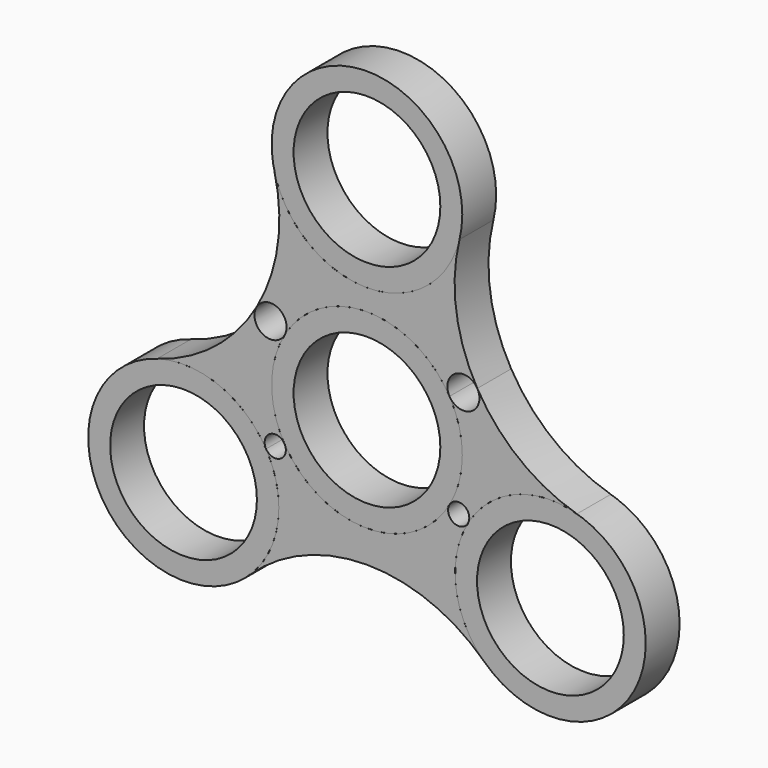
from build123d import *

# Parameters (mm, degrees)
F1_R     = 14.2875
F2_DEPTH = 6.35
F0_R     = 14.2875
F0_R_2   = 10.9982
F6_DEPTH = 25.4
F8_DEPTH = 25.4


with BuildPart() as f2:
    # F1 (on Front) → F2 (new body)
    with BuildSketch(Plane.XZ):
        with BuildLine():
            ThreePointArc((13.8718760728, 28.3289313848), (0, 17.4625), (-13.8718760728, 28.3289313848))
            ThreePointArc((-13.8718760728, 28.3289313848), (-16.5359438351, 9.5470316245), (-31.4695122777, -2.1510686152))
            ThreePointArc((-31.4695122777, -2.1510686152), (-18.912441482, -4.4535326513), (-13.2088065702, -15.875))
            ThreePointArc((-13.2088065702, -15.875), (-14.3517276668, -21.4743483284), (-17.5976362049, -26.1778627696))
            ThreePointArc((-17.5976362049, -26.1778627696), (0, -19.094063249), (17.5976362049, -26.1778627696))
            ThreePointArc((17.5976362049, -26.1778627696), (15.1229686136, -8.73125), (31.4695122777, -2.1510686152))
            ThreePointArc((31.4695122777, -2.1510686152), (16.5359438351, 9.5470316245), (13.8718760728, 28.3289313848))
        make_face()
        Circle(F1_R, mode=Mode.SUBTRACT)
    extrude(amount=F2_DEPTH)

    # F5 (on face) → F6 (cut)
    with BuildSketch(Plane.XZ.offset(6.35)):
        with BuildLine():
            ThreePointArc((12.3733379823, 7.1437499555), (15.0766559758, 6.02399903), (16.8579225203, 8.3453908122))
            ThreePointArc((16.8579225203, 8.3453908122), (16.7760327127, 8.9674057632), (16.535943943, 9.5470314377))
            ThreePointArc((16.535943943, 9.5470314377), (13.2530001547, 10.4266937926), (12.3733379823, 7.1437499555))
        make_face()
        with BuildLine():
            ThreePointArc((-16.5359438155, 9.5470316585), (-15.6562817429, 6.2640878931), (-12.3733379771, 7.1437499644))
            ThreePointArc((-12.3733379771, 7.1437499644), (-12.1332491122, 7.7233757372), (-12.0513592713, 8.3453908122))
            ThreePointArc((-12.0513592713, 8.3453908122), (-13.8326258217, 10.6667825961), (-16.5359438155, 9.5470316585))
        make_face()
    extrude(amount=-F6_DEPTH, mode=Mode.SUBTRACT)

    # F7 (on face) → F8 (cut)
    with BuildSketch(Plane.XZ.offset(6.35)):
        with BuildLine():
            ThreePointArc((15.1229686575, -8.731249924), (15.2815605457, -8.3483751917), (15.3356532851, -7.9375))
            ThreePointArc((15.3356532851, -7.9375), (14.1590284355, -6.4040927283), (12.3733378699, -7.1437501501))
            ThreePointArc((12.3733378699, -7.1437501501), (12.9544033981, -9.3123153938), (15.1229686575, -8.731249924))
        make_face()
        with BuildLine():
            ThreePointArc((-12.1606532851, -7.9375), (-12.2147460382, -7.5266247571), (-12.3733379657, -7.1437499842))
            ThreePointArc((-12.3733379657, -7.1437499842), (-14.5419032233, -6.5626846358), (-15.122968694, -8.7312498607))
            ThreePointArc((-15.122968694, -8.7312498607), (-13.3372781286, -9.47090727), (-12.1606532851, -7.9375))
        make_face()
    extrude(amount=-F8_DEPTH, mode=Mode.SUBTRACT)


with BuildPart() as f2b:
    # F0 (on Front) → F2, piece 2 (new body)
    with BuildSketch(Plane.XZ):
        with Locations((0, 31.75)):
            Circle(F0_R)
        with Locations((0, 31.75)):
            Circle(F0_R_2, mode=Mode.SUBTRACT)
    extrude(amount=F2_DEPTH)


with BuildPart() as f2c:
    # F0 (on Front) → F2, piece 3 (new body)
    with BuildSketch(Plane.XZ):
        with Locations((-27.4963065702, -15.875)):
            Circle(F0_R)
        with Locations((-27.4963065702, -15.875)):
            Circle(F0_R_2, mode=Mode.SUBTRACT)
    extrude(amount=F2_DEPTH)


with BuildPart() as f2d:
    # F0 (on Front) → F2, piece 4 (new body)
    with BuildSketch(Plane.XZ):
        with Locations((27.4963065702, -15.875)):
            Circle(F0_R)
        with Locations((27.4963065702, -15.875)):
            Circle(F0_R_2, mode=Mode.SUBTRACT)
    extrude(amount=F2_DEPTH)


with BuildPart() as f2e:
    # F0 (on Front) → F2, piece 5 (new body)
    with BuildSketch(Plane.XZ):
        Circle(F0_R)
        Circle(F0_R_2, mode=Mode.SUBTRACT)
    extrude(amount=F2_DEPTH)


solid = Compound([f2.part, f2b.part, f2c.part, f2d.part, f2e.part])
